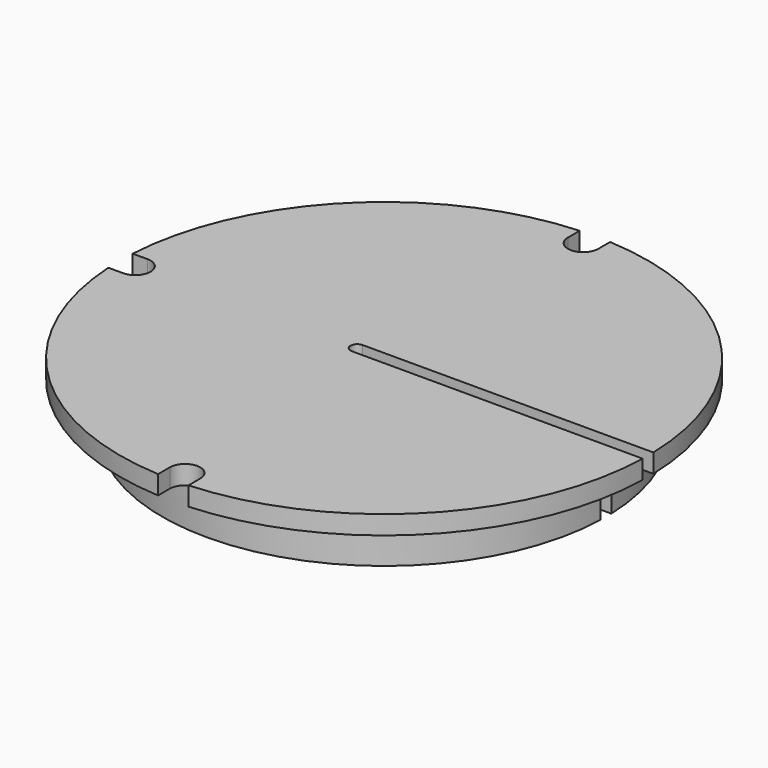
from build123d import *

# Parameters (mm, degrees)
F0_R            = 29.5
F2_DEPTH        = 2.1
F4_DEPTH        = 2.1
F4_COPIES_COUNT = 3
F4_COPIES_ANGLE = 180
F6_DEPTH        = 2.1
F8_DEPTH        = 5.45


# Not quite as in the source:
# - a pattern or mirror of a feature is missing from the dataset's text; its kind, count and spacing are read off the source's solid


with BuildPart() as f2:
    # F0 (on Top) → F2 (new body)
    with BuildSketch(Plane.XY):
        Circle(F0_R)
    extrude(amount=F2_DEPTH)

    # F3 (on face) → F4 (cut, through all)
    with BuildSketch(Plane.XY.offset(2.1)):
        with BuildLine():
            ThreePointArc((-1.7, 27.8), (0, 26.1), (1.7, 27.8))
            Line((1.7, 27.8), (1.7, 29.4509762147))
            ThreePointArc((1.7, 29.4509762147), (0, 29.5), (-1.7, 29.4509762147))
            Line((-1.7, 29.4509762147), (-1.7, 27.8))
        make_face()
    f4 = extrude(amount=-F4_DEPTH, mode=Mode.SUBTRACT)

    # F4_copies: F4 ×3 about axis
    f4_copies_axis = Axis((0, 0, 0), (0, 0, 1))
    for i in range(1, F4_COPIES_COUNT):
        add(f4.rotate(f4_copies_axis, i * F4_COPIES_ANGLE / (F4_COPIES_COUNT - 1)), mode=Mode.SUBTRACT)

    # F5 (on face) → F6 (cut, through all)
    with BuildSketch(Plane.XY.offset(2.1)):
        with BuildLine():
            ThreePointArc((-3, 0.75), (-3.75, 0), (-3, -0.75))
            Line((-3, -0.75), (29.4904645606, -0.75))
            ThreePointArc((29.4904645606, -0.75), (29.5, 0), (29.4904645606, 0.75))
            Line((29.4904645606, 0.75), (-3, 0.75))
        make_face()
    extrude(amount=-F6_DEPTH, mode=Mode.SUBTRACT)

    # F7 (on face) → F8 (join)
    with BuildSketch(Plane(origin=(0, 0, 0), x_dir=(1, 0, 0), z_dir=(0, 0, -1))):
        with BuildLine():
            Line((22.9877684867, 0.75), (24.78865668, 0.75))
            ThreePointArc((24.78865668, 0.75), (-24.8, 0), (24.78865668, -0.75))
            Line((24.78865668, -0.75), (22.9877684867, -0.75))
            ThreePointArc((22.9877684867, -0.75), (-23, 0), (22.9877684867, 0.75))
        make_face()
    extrude(amount=F8_DEPTH)


solid = f2.part
